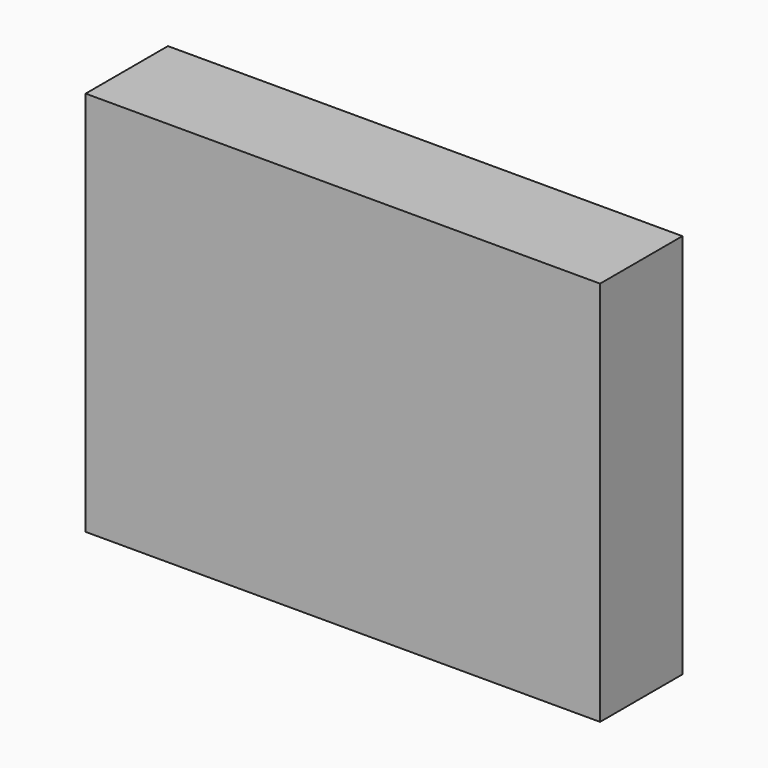
from build123d import *

# Parameters (mm, degrees)
F4_DEPTH = 6.35


# Not quite as in the source:
# - the program builds the solid bodies; features that only make, move or delete a surface that nothing else refers to are left out


with BuildPart() as f4:
    # F0 (on Front) → F4 (new body)
    with BuildSketch(Plane.XZ):
        Polygon((12.5453299433, 15.9246460537), (-19.2046700567, 15.9246460537), (-19.2046700567, -7.8878539463), (12.5453299433, -7.8878539463), (12.5453299433, -6.3003510131), (12.5453299433, -4.7128512226), (12.5453299433, -3.1253514321), (12.5453299433, -1.5378516416), (12.5453299433, 0.0496481488), (12.5453299433, 1.6371479393), (12.5453299433, 3.2246477298), (12.5453299433, 4.8121475203), (12.5453299433, 6.3996473108), (12.5453299433, 7.9871471013), (12.5453299433, 9.5746468917), (12.5453299433, 11.1621466822), (12.5453299433, 12.7496464727), (12.5453299433, 14.3371462632), align=None)
    extrude(amount=F4_DEPTH)


solid = f4.part
